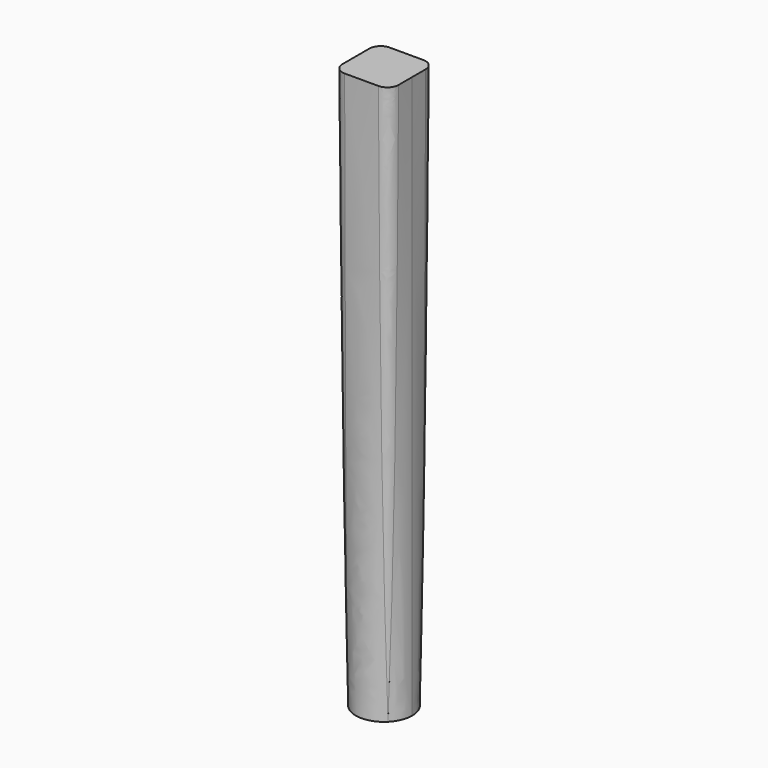
from build123d import *

# Parameters (mm, degrees)
F0_R = 25
F2_W = 50
F2_H = 50
F4_R = 10


with BuildPart() as f3:
    # F0 (on Top) → F3 section 0
    with BuildSketch(Plane.XY):
        Circle(F0_R)
    # F2 (on offset) → F3 section 1
    with BuildSketch(Plane.XY.offset(500)):
        Rectangle(F2_W, F2_H)
    loft()

    # F4
    f4_edges = [f3.edges().sort_by_distance(p)[0] for p in [
        (21.338835, 21.338835, 250),
        (-21.338835, 21.338835, 250),
        (-21.338835, -21.338835, 250),
        (21.338835, -21.338835, 250),
    ]]
    fillet(f4_edges, radius=F4_R)


solid = f3.part
